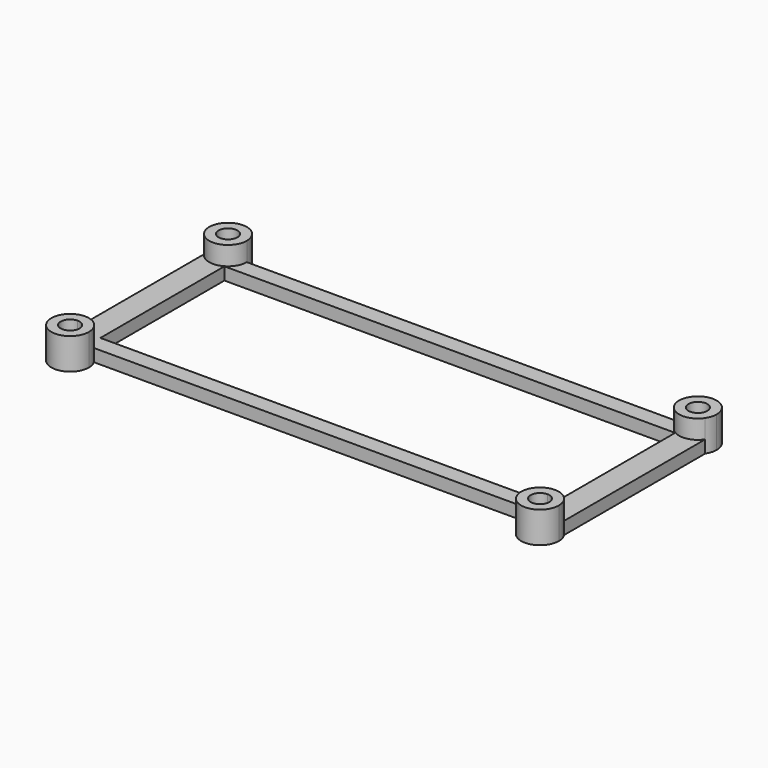
from build123d import *
from build123d import SkipClean  # not in build123d's __all__

# Parameters (mm, degrees)
F0_W     = 71.95
F0_H     = 24.75
F1_DEPTH = 2
F2_DEPTH = 5


with BuildPart() as f1:
    # F0 (on Top) → F1 (new body)
    with BuildSketch(Plane.XY):
        with BuildLine():
            Line((34.5, 15), (-34.5, 15))
            ThreePointArc((-34.5, 15), (-36.6339745962, 12.1277186767), (-40, 13.3416876048))
            Line((-40, 13.3416876048), (-40, -14.8416876048))
            ThreePointArc((-40, -14.8416876048), (-37.4068848056, -13.5014454214), (-34.9019237886, -15))
            Line((-34.9019237886, -15), (34.9019237886, -15))
            ThreePointArc((34.9019237886, -15), (37.4068848056, -13.5014454214), (40, -14.8416876048))
            Line((40, -14.8416876048), (40, 13.3416876048))
            ThreePointArc((40, 13.3416876048), (36.6339745962, 12.1277186767), (34.5, 15))
        make_face()
        Rectangle(F0_W, F0_H, mode=Mode.SUBTRACT)
        with BuildLine():
            Line((-34.5, 15), (-36, 15))
            ThreePointArc((-36, 15), (-37.5, 13.5), (-39, 15))
            Line((-39, 15), (-40, 15))
            Line((-40, 15), (-40, 13.3416876048))
            ThreePointArc((-40, 13.3416876048), (-36.6339745962, 12.1277186767), (-34.5, 15))
        make_face()
        with BuildLine():
            Line((36, 15), (34.5, 15))
            ThreePointArc((34.5, 15), (36.6339745962, 12.1277186767), (40, 13.3416876048))
            Line((40, 13.3416876048), (40, 15))
            Line((40, 15), (39, 15))
            ThreePointArc((39, 15), (37.5, 13.5), (36, 15))
        make_face()
        with BuildLine():
            Line((40, -15), (40, -14.8416876048))
            ThreePointArc((40, -14.8416876048), (37.4068848056, -13.5014454214), (34.9019237886, -15))
            Line((34.9019237886, -15), (37.5, -15))
            Line((37.5, -15), (40, -15))
        make_face()
        with BuildLine():
            ThreePointArc((-34.9019237886, -15), (-37.4068848056, -13.5014454214), (-40, -14.8416876048))
            Line((-40, -14.8416876048), (-40, -15))
            Line((-40, -15), (-37.5, -15))
            Line((-37.5, -15), (-34.9019237886, -15))
        make_face()
    extrude(amount=F1_DEPTH)

    # F0 (on Top) → F2 (join)
    with BuildSketch(Plane.XY):
        with BuildLine():
            Line((-34.5, 15), (-36, 15))
            ThreePointArc((-36, 15), (-37.5, 13.5), (-39, 15))
            Line((-39, 15), (-40, 15))
            Line((-40, 15), (-40, 13.3416876048))
            ThreePointArc((-40, 13.3416876048), (-36.6339745962, 12.1277186767), (-34.5, 15))
        make_face()
        with BuildLine():
            ThreePointArc((-39, 15), (-37.5, 16.5), (-36, 15))
            Line((-36, 15), (-34.5, 15))
            ThreePointArc((-34.5, 15), (-38.3660254038, 17.8722813233), (-40, 13.3416876048))
            Line((-40, 13.3416876048), (-40, 15))
            Line((-40, 15), (-39, 15))
        make_face()
        with BuildLine():
            Line((-40, -15), (-40, -14.8416876048))
            ThreePointArc((-40, -14.8416876048), (-38.3660254038, -19.3722813233), (-34.5, -16.5))
            ThreePointArc((-34.5, -16.5), (-34.6022225211, -15.7235428647), (-34.9019237886, -15))
            Line((-34.9019237886, -15), (-37.5, -15))
            Line((-37.5, -15), (-40, -15))
        make_face()
        with BuildLine():
            ThreePointArc((-36, -16.5), (-38.5606601718, -17.5606601718), (-37.5, -15))
            ThreePointArc((-37.5, -15), (-36.4393398282, -15.4393398282), (-36, -16.5))
        make_face(mode=Mode.SUBTRACT)
        with BuildLine():
            ThreePointArc((-34.9019237886, -15), (-37.4068848056, -13.5014454214), (-40, -14.8416876048))
            Line((-40, -14.8416876048), (-40, -15))
            Line((-40, -15), (-37.5, -15))
            Line((-37.5, -15), (-34.9019237886, -15))
        make_face()
        with BuildLine():
            ThreePointArc((40.5, -16.5), (40.3722813233, -15.6339745962), (40, -14.8416876048))
            Line((40, -14.8416876048), (40, -15))
            Line((40, -15), (37.5, -15))
            Line((37.5, -15), (34.9019237886, -15))
            ThreePointArc((34.9019237886, -15), (36.7235428647, -19.3977774789), (40.5, -16.5))
        make_face()
        with BuildLine():
            ThreePointArc((39, -16.5), (36.4393398282, -17.5606601718), (37.5, -15))
            ThreePointArc((37.5, -15), (38.5606601718, -15.4393398282), (39, -16.5))
        make_face(mode=Mode.SUBTRACT)
        with BuildLine():
            Line((40, -15), (40, -14.8416876048))
            ThreePointArc((40, -14.8416876048), (37.4068848056, -13.5014454214), (34.9019237886, -15))
            Line((34.9019237886, -15), (37.5, -15))
            Line((37.5, -15), (40, -15))
        make_face()
        with BuildLine():
            ThreePointArc((40.5, 15), (37.5, 18), (34.5, 15))
            Line((34.5, 15), (36, 15))
            ThreePointArc((36, 15), (37.5, 16.5), (39, 15))
            Line((39, 15), (40, 15))
            Line((40, 15), (40, 13.3416876048))
            ThreePointArc((40, 13.3416876048), (40.3722813233, 14.1339745962), (40.5, 15))
        make_face()
        with BuildLine():
            Line((36, 15), (34.5, 15))
            ThreePointArc((34.5, 15), (36.6339745962, 12.1277186767), (40, 13.3416876048))
            Line((40, 13.3416876048), (40, 15))
            Line((40, 15), (39, 15))
            ThreePointArc((39, 15), (37.5, 13.5), (36, 15))
        make_face()
    with SkipClean():  # cleaning this boolean's faces spoils the solid; the shape is the same uncleaned
        extrude(amount=F2_DEPTH)


solid = f1.part
